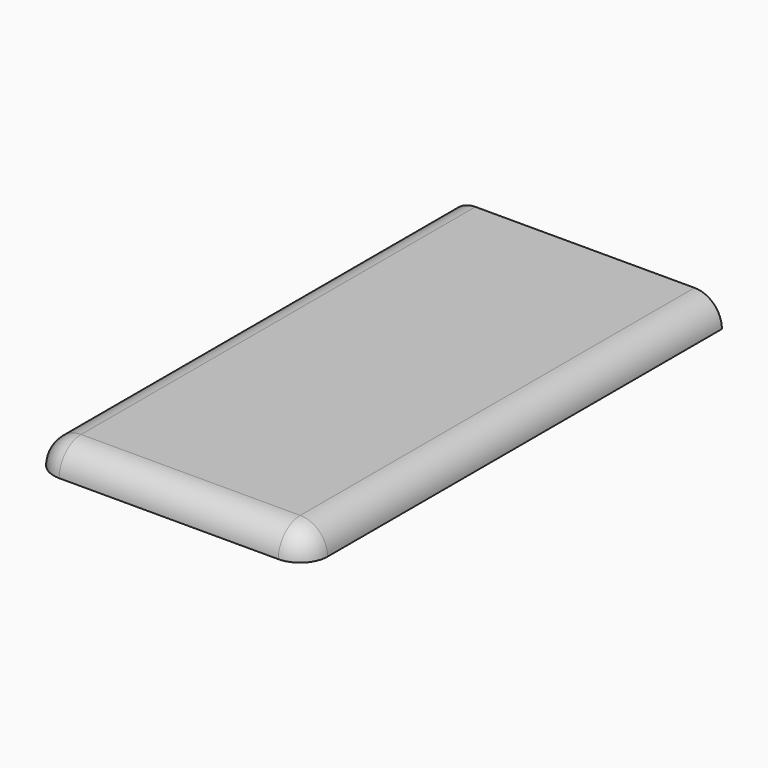
from build123d import *

# Parameters (mm, degrees)
F0_W     = 40
F0_H     = 76
F1_DEPTH = 4
F2_R     = 3.99999


# Not quite as in the source:
# - a fillet or chamfer is up to 0.001 mm smaller than in the source, because OpenCascade refuses the exact size


with BuildPart() as f1:
    # F0 (on Top) → F1 (new body)
    with BuildSketch(Plane.XY):
        with Locations((20, 38)):
            Rectangle(F0_W, F0_H)
    extrude(amount=F1_DEPTH)

    # F2 (radius 4 in the source; OpenCascade refuses exactly that, so slightly less here)
    f2_edges = [f1.edges().sort_by_distance(p)[0] for p in [
        (40, 38, 4),
        (20, 0, 4),
        (0, 38, 4),
        (40, 0, 2),
        (0, 0, 2),
    ]]
    fillet(f2_edges, radius=F2_R)


solid = f1.part
